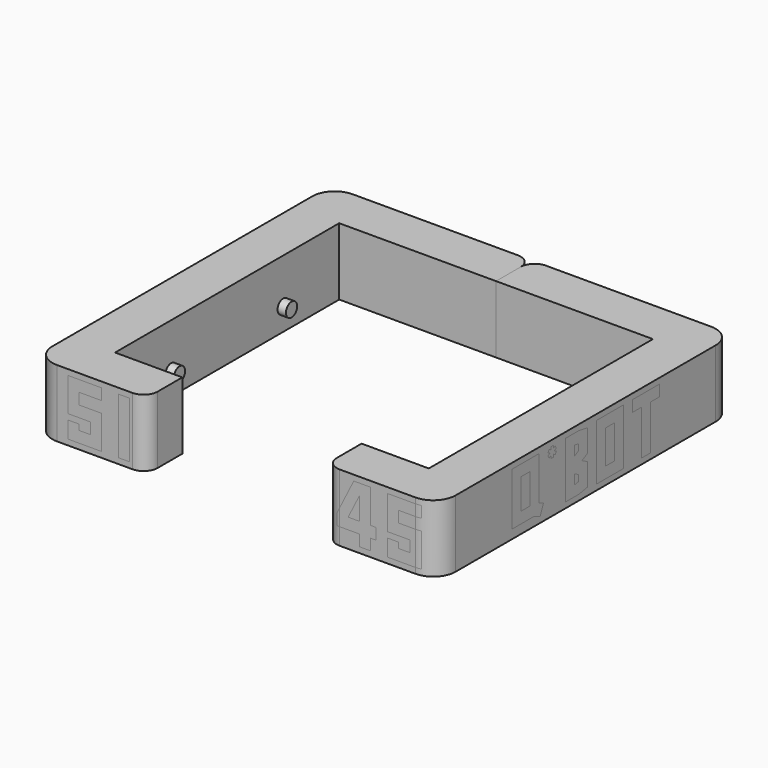
from build123d import *

# Parameters (mm, degrees)
F1_DEPTH       = 15.24
F2_R           = 1.5875
F3_DEPTH       = 1.905
F5_DEPTH       = 15.24
F6_R           = 1.5875
F7_DEPTH       = 1.905
F9_DEPTH       = 0.79375
F10_W          = 2.54
F10_H          = 12.7
F11_DEPTH      = 0.79375
F12_W          = 2.54
F12_H          = 12.7
F13_DEPTH      = 0.79375
F14_W          = 2.54
F14_H          = 12.7
F15_DEPTH      = 0.79375
F17_DEPTH      = 0.79375
F18_R          = 5.08
F19_T1_DEPTH   = 40.64
F20_T1_DEPTH   = 31.115
F20_2_T1_DEPTH = 31.115
F21_DEPTH      = 0.79375
F22_DEPTH      = 0.79375
F23_DEPTH      = 0.79375
F25_DEPTH      = 25.4
F27_DEPTH      = 25.4
F29_DEPTH      = 25.4
F30_W          = 2.54
F30_H          = 6.8751920004
F30_W_2        = 7.62
F30_H_2        = 12.7
F30_H_3        = 7.62
F31_DEPTH      = 0.79375
F32_DEPTH      = 0.79375


# Not quite as in the source:
# - a fillet or chamfer that OpenCascade refuses, or shapes differently, is made with other operations: its cross-section is extruded or revolved along the edge and cut away or added


with BuildPart() as f1:
    # F0 (on Top) → F1 (new body)
    with BuildSketch(Plane.XY):
        Polygon((0, 38.8312135783), (0, 28.6712135783), (35.56, 28.6712135783), (35.56, -34.8287864217), (20.32, -34.8287864217), (20.32, -44.9887864217), (45.72, -44.9887864217), (45.72, 38.8312135783), align=None)
    extrude(amount=F1_DEPTH)

    # F2 (on face) → F3 (join)
    with BuildSketch(Plane(origin=(35.56, 0, 0), x_dir=(0, -1, 0), z_dir=(-1, 0, 0))):
        with Locations((-12.7962135783, 5.08)):
            Circle(F2_R)
        with Locations((18.9537864217, 5.08)):
            Circle(F2_R)
    extrude(amount=F3_DEPTH)

    # F8 (on face) → F9 (cut)
    with BuildSketch(Plane.XZ.offset(44.9887864217)):
        Polygon((26.67, 13.97), (22.86, 6.35), (22.86, 3.81), (27.94, 3.81), (27.94, 1.27), (30.48, 1.27), (30.48, 3.81), (31.75, 3.81), (31.75, 6.35), (30.48, 6.35), (30.48, 13.97), align=None)
        Polygon((27.94, 11.43), (27.94, 6.35), (25.4, 6.35), align=None, mode=Mode.SUBTRACT)
        Polygon((41.91, 11.43), (41.91, 13.97), (34.29, 13.97), (34.29, 6.35), (39.37, 6.35), (39.37, 3.81), (36.83, 3.81), (36.83, 5.08), (34.29, 5.08), (34.29, 1.27), (41.91, 1.27), (41.91, 8.89), (36.83, 8.89), (36.83, 11.43), align=None)
    extrude(amount=-F9_DEPTH, mode=Mode.SUBTRACT)

    # F14 (on face) → F15 (cut)
    with BuildSketch(Plane(origin=(0, 38.8312135783, 0), x_dir=(-1, 0, 0), z_dir=(0, 1, 0))):
        Polygon((-8.89, 11.43), (-8.89, 13.97), (-16.51, 13.97), (-16.51, 6.35), (-11.43, 6.35), (-11.43, 3.81), (-13.97, 3.81), (-13.97, 5.08), (-16.51, 5.08), (-16.51, 1.27), (-8.89, 1.27), (-8.89, 8.89), (-13.97, 8.89), (-13.97, 11.43), align=None)
        with Locations((-5.08, 7.62)):
            Rectangle(F14_W, F14_H)
    extrude(amount=-F15_DEPTH, mode=Mode.SUBTRACT)

    # F19: fillet of radius 5.08 on 2 edges, made by hand

    # F19_s2 → F19_t1 (cut)
    with BuildSketch(Plane.XY.offset(-12.7)):
        with BuildLine():
            ThreePointArc((45.72, -39.9087864217), (44.2321024484, -43.5008888701), (40.64, -44.9887864217))
            Line((40.64, -44.9887864217), (45.72, -44.9887864217))
            Line((45.72, -44.9887864217), (45.72, -39.9087864217))
        make_face()
        with BuildLine():
            ThreePointArc((40.64, 38.8312135783), (44.2321024484, 37.3433160267), (45.72, 33.7512135783))
            Line((45.72, 33.7512135783), (45.72, 38.8312135783))
            Line((45.72, 38.8312135783), (40.64, 38.8312135783))
        make_face()
    extrude(amount=F19_T1_DEPTH, mode=Mode.SUBTRACT)

    # F20: fillet of radius 3.175 on 2 edges, made by hand

    # F20_s2 → F20_t1 (cut)
    with BuildSketch(Plane.XY.offset(-7.9375)):
        with BuildLine():
            ThreePointArc((23.495, -44.9887864217), (21.2499359697, -44.058850452), (20.32, -41.8137864217))
            Line((20.32, -41.8137864217), (20.32, -44.9887864217))
            Line((20.32, -44.9887864217), (23.495, -44.9887864217))
        make_face()
        with BuildLine():
            ThreePointArc((0, 35.6562135783), (0.9299359697, 37.9012776086), (3.175, 38.8312135783))
            Line((3.175, 38.8312135783), (0, 38.8312135783))
            Line((0, 38.8312135783), (0, 35.6562135783))
        make_face()
    extrude(amount=F20_T1_DEPTH, mode=Mode.SUBTRACT)


with BuildPart() as f5:
    # F4 (on Top) → F5 (new body)
    with BuildSketch(Plane.XY):
        Polygon((-35.56, 28.6712135783), (0, 28.6712135783), (0, 38.8312135783), (-45.72, 38.8312135783), (-45.72, -44.9887864217), (-20.32, -44.9887864217), (-20.32, -34.8287864217), (-35.56, -34.8287864217), align=None)
    extrude(amount=F5_DEPTH)

    # F6 (on face) → F7 (join)
    with BuildSketch(Plane.YZ.offset(-35.56)):
        with Locations((12.7962135783, 5.08)):
            Circle(F6_R)
        with Locations((-18.9537864217, 5.08)):
            Circle(F6_R)
    extrude(amount=F7_DEPTH)

    # F10 (on face) → F11 (cut)
    with BuildSketch(Plane.XZ.offset(44.9887864217)):
        Polygon((-30.48, 11.43), (-30.48, 13.97), (-38.1, 13.97), (-38.1, 6.35), (-33.02, 6.35), (-33.02, 3.81), (-35.56, 3.81), (-35.56, 5.08), (-38.1, 5.08), (-38.1, 1.27), (-30.48, 1.27), (-30.48, 8.89), (-35.56, 8.89), (-35.56, 11.43), align=None)
        with Locations((-25.4, 7.62)):
            Rectangle(F10_W, F10_H)
    extrude(amount=-F11_DEPTH, mode=Mode.SUBTRACT)

    # F12 (on face) → F13 (cut)
    with BuildSketch(Plane(origin=(-45.72, 0, 0), x_dir=(0, -1, 0), z_dir=(-1, 0, 0))):
        Polygon((-6.4462135783, 11.43), (-6.4462135783, 13.97), (-14.0662135783, 13.97), (-14.0662135783, 6.35), (-8.9862135783, 6.35), (-8.9862135783, 3.81), (-11.5262135783, 3.81), (-11.5262135783, 5.08), (-14.0662135783, 5.08), (-14.0662135783, 1.27), (-6.4462135783, 1.27), (-6.4462135783, 8.89), (-11.5262135783, 8.89), (-11.5262135783, 11.43), align=None)
        with Locations((-2.6362135783, 7.62)):
            Rectangle(F12_W, F12_H)
        Polygon((8.7937864217, 13.97), (4.9837864217, 13.97), (1.1737864217, 6.35), (1.1737864217, 3.81), (6.2537864217, 3.81), (6.2537864217, 1.27), (8.7937864217, 1.27), (8.7937864217, 3.81), (10.0637864217, 3.81), (10.0637864217, 6.35), (8.7937864217, 6.35), align=None)
        Polygon((6.2537864217, 11.43), (6.2537864217, 6.35), (3.7137864217, 6.35), align=None, mode=Mode.SUBTRACT)
        Polygon((20.2237864217, 11.43), (20.2237864217, 13.97), (12.6037864217, 13.97), (12.6037864217, 6.35), (17.6837864217, 6.35), (17.6837864217, 3.81), (15.1437864217, 3.81), (15.1437864217, 5.08), (12.6037864217, 5.08), (12.6037864217, 1.27), (20.2237864217, 1.27), (20.2237864217, 8.89), (15.1437864217, 8.89), (15.1437864217, 11.43), align=None)
    extrude(amount=-F13_DEPTH, mode=Mode.SUBTRACT)

    # F16 (on face) → F17 (cut)
    with BuildSketch(Plane(origin=(0, 38.8312135783, 0), x_dir=(-1, 0, 0), z_dir=(0, 1, 0))):
        Polygon((6.35, 13.97), (2.54, 6.35), (2.54, 3.81), (7.62, 3.81), (7.62, 1.27), (10.16, 1.27), (10.16, 3.81), (11.43, 3.81), (11.43, 6.35), (10.16, 6.35), (10.16, 13.97), align=None)
        Polygon((7.62, 11.43), (7.62, 6.35), (5.08, 6.35), align=None, mode=Mode.SUBTRACT)
        Polygon((21.59, 11.43), (21.59, 13.97), (13.97, 13.97), (13.97, 6.35), (19.05, 6.35), (19.05, 3.81), (16.51, 3.81), (16.51, 5.08), (13.97, 5.08), (13.97, 1.27), (21.59, 1.27), (21.59, 8.89), (16.51, 8.89), (16.51, 11.43), align=None)
    extrude(amount=-F17_DEPTH, mode=Mode.SUBTRACT)

    # F18
    f18_edges = [f5.edges().sort_by_distance(p)[0] for p in [
        (-45.72, 38.831214, 7.62),
        (-45.72, -44.988786, 7.62),
    ]]
    fillet(f18_edges, radius=F18_R)

    # F20#2: fillet of radius 3.175 on 2 edges, made by hand

    # F20_2_s2 → F20_2_t1 (cut)
    with BuildSketch(Plane.XY.offset(-7.9375)):
        with BuildLine():
            ThreePointArc((-23.495, -44.9887864217), (-21.2499359697, -44.058850452), (-20.32, -41.8137864217))
            Line((-20.32, -41.8137864217), (-20.32, -44.9887864217))
            Line((-20.32, -44.9887864217), (-23.495, -44.9887864217))
        make_face()
        with BuildLine():
            ThreePointArc((-3.175, 38.8312135783), (-0.9299359697, 37.9012776086), (0, 35.6562135783))
            Line((0, 35.6562135783), (0, 38.8312135783))
            Line((0, 38.8312135783), (-3.175, 38.8312135783))
        make_face()
    extrude(amount=F20_2_T1_DEPTH, mode=Mode.SUBTRACT)


with BuildPart() as f21:
    # F21 (new): a face of the model
    f21_faces = [f1.part.faces().sort_by_distance(p)[0] for p in [
        (24.9036570157, -44.1950364217, 10.0906714922),
    ]]
    extrude(f21_faces, amount=F21_DEPTH)

    # F26 (on face) → F27 (cut)
    with BuildSketch(Plane(origin=(0, 0, 3.81), x_dir=(1, 0, 0), z_dir=(0, 0, -1))):
        with BuildLine():
            ThreePointArc((22.86, 44.924638395), (23.1758840456, 44.9727087075), (23.495, 44.9887864217))
            Line((23.495, 44.9887864217), (22.86, 44.9887864217))
            Line((22.86, 44.9887864217), (22.86, 44.924638395))
        make_face()
    extrude(amount=-F27_DEPTH, mode=Mode.SUBTRACT)


with BuildPart() as f21b:
    # F21#2 (new): a face of the model
    f21_2_faces = [f1.part.faces().sort_by_distance(p)[0] for p in [
        (37.9895652174, -44.1950364217, 7.4819565217),
    ]]
    extrude(f21_2_faces, amount=F21_DEPTH)

    # F24 (on face) → F25 (cut)
    with BuildSketch(Plane(origin=(0, 0, 1.27), x_dir=(1, 0, 0), z_dir=(0, 0, -1))):
        with BuildLine():
            ThreePointArc((40.64, 44.9887864217), (41.2801018058, 44.9482972787), (41.91, 44.8274752714))
            Line((41.91, 44.8274752714), (41.91, 44.9887864217))
            Line((41.91, 44.9887864217), (40.64, 44.9887864217))
        make_face()
    extrude(amount=-F25_DEPTH, mode=Mode.SUBTRACT)


with BuildPart() as f21c:
    # F21#3 (new): a face of the model
    f21_3_faces = [f5.part.faces().sort_by_distance(p)[0] for p in [
        (-25.4, -44.1950364217, 7.62),
    ]]
    extrude(f21_3_faces, amount=F21_DEPTH)


with BuildPart() as f21d:
    # F21#4 (new): a face of the model
    f21_4_faces = [f5.part.faces().sort_by_distance(p)[0] for p in [
        (-34.4004347826, -44.1950364217, 7.4819565217),
    ]]
    extrude(f21_4_faces, amount=F21_DEPTH)


with BuildPart() as f22:
    # F22 (new): a face of the model
    f22_faces = [f5.part.faces().sort_by_distance(p)[0] for p in [
        (-44.92625, 10.3666483609, 7.4819565217),
    ]]
    extrude(f22_faces, amount=F22_DEPTH)


with BuildPart() as f22b:
    # F22#2 (new): a face of the model
    f22_2_faces = [f5.part.faces().sort_by_distance(p)[0] for p in [
        (-44.92625, 2.6362135783, 7.62),
    ]]
    extrude(f22_2_faces, amount=F22_DEPTH)


with BuildPart() as f22c:
    # F22#3 (new): a face of the model
    f22_3_faces = [f5.part.faces().sort_by_distance(p)[0] for p in [
        (-44.92625, -9.4287864217, 3.9650232563),
    ]]
    extrude(f22_3_faces, amount=F22_DEPTH)


with BuildPart() as f22d:
    # F22#4 (new): a face of the model
    f22_4_faces = [f5.part.faces().sort_by_distance(p)[0] for p in [
        (-44.92625, -16.3033516391, 7.4819565217),
    ]]
    extrude(f22_4_faces, amount=F22_DEPTH)


with BuildPart() as f23:
    # F23 (new): a face of the model
    f23_faces = [f1.part.faces().sort_by_distance(p)[0] for p in [
        (12.8104347826, 38.0374635783, 7.4819565217),
    ]]
    extrude(f23_faces, amount=F23_DEPTH)


with BuildPart() as f23b:
    # F23#2 (new): a face of the model
    f23_2_faces = [f1.part.faces().sort_by_distance(p)[0] for p in [
        (5.08, 38.0374635783, 7.62),
    ]]
    extrude(f23_2_faces, amount=F23_DEPTH)


with BuildPart() as f23c:
    # F23#3 (new): a face of the model
    f23_3_faces = [f5.part.faces().sort_by_distance(p)[0] for p in [
        (-4.5836570157, 38.0374635783, 10.0906714922),
    ]]
    extrude(f23_3_faces, amount=F23_DEPTH)

    # F28 (on face) → F29 (cut)
    with BuildSketch(Plane(origin=(0, 0, 3.81), x_dir=(1, 0, 0), z_dir=(0, 0, -1))):
        with BuildLine():
            ThreePointArc((-2.54, -38.7670655516), (-2.8558840456, -38.8151358641), (-3.175, -38.8312135783))
            Line((-3.175, -38.8312135783), (-2.54, -38.8312135783))
            Line((-2.54, -38.8312135783), (-2.54, -38.7670655516))
        make_face()
    extrude(amount=-F29_DEPTH, mode=Mode.SUBTRACT)


with BuildPart() as f23d:
    # F23#4 (new): a face of the model
    f23_4_faces = [f5.part.faces().sort_by_distance(p)[0] for p in [
        (-17.6695652174, 38.0374635783, 7.4819565217),
    ]]
    extrude(f23_4_faces, amount=F23_DEPTH)


with BuildPart() as f1_1:
    add(f1.part)

    # F30 (on face) → F31 (cut)
    with BuildSketch(Plane.YZ.offset(45.72)):
        Polygon((-16.3094183994, 13.97), (-23.9294183994, 13.97), (-23.9294183994, 2.0148079996), (-17.7994728489, 2.0148079996), (-16.0202090098, 1.27), (-15.0394183994, 3.6130001662), (-16.3094183994, 4.1446279881), align=None)
        with Locations((-20.1194183994, 7.9924039998)):
            Rectangle(F30_W, F30_H, mode=Mode.SUBTRACT)
        Polygon((-11.949492268, 12.7850738686), (-11.3995661366, 13.1025738686), (-11.7170661366, 13.6525), (-12.266992268, 13.335), (-12.266992268, 13.97), (-12.901992268, 13.97), (-12.901992268, 13.335), (-13.4519183994, 13.6525), (-13.7694183994, 13.1025738686), (-13.219492268, 12.7850738686), (-13.7694183994, 12.4675738686), (-13.4519183994, 11.9176477372), (-12.901992268, 12.2351477372), (-12.901992268, 11.6001477372), (-12.266992268, 11.6001477372), (-12.266992268, 12.2351477372), (-11.7170661366, 11.9176477372), (-11.3995661366, 12.4675738686), align=None)
        Polygon((-5.0495661366, 13.97), (-8.8595661366, 13.97), (-8.8595661366, 1.27), (-5.0495661366, 1.27), (-2.548154444, 1.7110663713), (-2.548154444, 6.7910663713), (-4.1484195331, 7.62), (-2.548154444, 8.4489336287), (-2.548154444, 13.5289336287), align=None)
        Polygon((-6.3195661366, 3.6252483287), (-6.3195661366, 5.8841063813), (-5.088154444, 5.246237962), (-5.088154444, 3.8423794345), align=None, mode=Mode.SUBTRACT)
        Polygon((-6.3195661366, 9.3558936187), (-6.3195661366, 11.6147516713), (-5.088154444, 11.3976205655), (-5.088154444, 9.993762038), align=None, mode=Mode.SUBTRACT)
        with Locations((3.801845556, 7.62)):
            Rectangle(F30_W_2, F30_H_2)
        with Locations((3.801845556, 7.62)):
            Rectangle(F30_W, F30_H_3, mode=Mode.SUBTRACT)
        Polygon((17.771845556, 13.97), (10.151845556, 13.97), (10.151845556, 11.43), (12.691845556, 11.43), (12.691845556, 1.27), (15.231845556, 1.27), (15.231845556, 11.43), (17.771845556, 11.43), align=None)
    extrude(amount=-F31_DEPTH, mode=Mode.SUBTRACT)


with BuildPart() as f32:
    # F32 (new): a face of the model
    f32_faces = [f1_1.part.faces().sort_by_distance(p)[0] for p in [
        (44.92625, -16.8499805537, 1.785403809),
    ]]
    extrude(f32_faces, amount=F32_DEPTH)


with BuildPart() as f32b:
    # F32#2 (new): a face of the model
    f32_2_faces = [f1_1.part.faces().sort_by_distance(p)[0] for p in [
        (44.92625, -12.584492268, 12.7850738686),
    ]]
    extrude(f32_2_faces, amount=F32_DEPTH)


with BuildPart() as f32c:
    # F32#3 (new): a face of the model
    f32_3_faces = [f1_1.part.faces().sort_by_distance(p)[0] for p in [
        (44.92625, -5.7834089461, 7.62),
    ]]
    extrude(f32_3_faces, amount=F32_DEPTH)


with BuildPart() as f32d:
    # F32#4 (new): a face of the model
    f32_4_faces = [f1_1.part.faces().sort_by_distance(p)[0] for p in [
        (44.92625, 0.1399517342, 7.62),
    ]]
    extrude(f32_4_faces, amount=F32_DEPTH)


with BuildPart() as f32e:
    # F32#5 (new): a face of the model
    f32_5_faces = [f1_1.part.faces().sort_by_distance(p)[0] for p in [
        (44.92625, 13.961845556, 9.0714285714),
    ]]
    extrude(f32_5_faces, amount=F32_DEPTH)


solid = Compound([f5.part, f21.part, f21b.part, f21c.part, f21d.part, f22.part, f22b.part, f22c.part, f22d.part, f23.part, f23b.part, f23c.part, f23d.part, f1_1.part, f32.part, f32b.part, f32c.part, f32d.part, f32e.part])
